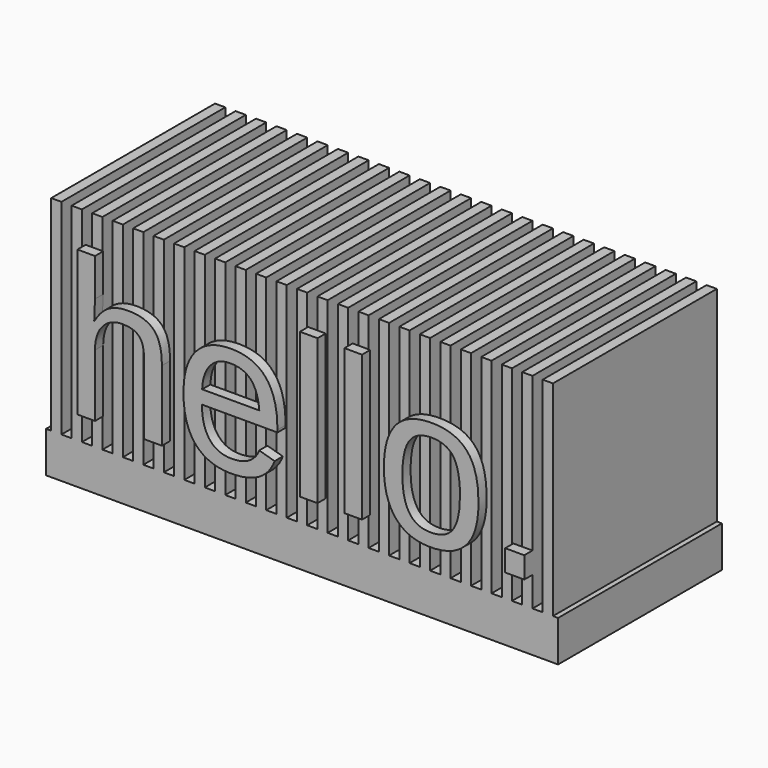
from build123d import *

# Parameters (mm, degrees)
F0_W         = 63.5
F0_H         = 25.4
F1_DEPTH     = 5.08
F2_W         = 1.27
F2_H         = 25.4
F3_DEPTH     = 25.4
F4_TEXT_SIZE = 24.8562691131
F5_DEPTH     = 1.27


# Not quite as in the source:
# - Text() gives the source's letters only with a copy of the font that has no kerning and outlines rounded to 1/6400 em; it was checked with that copy


with BuildPart() as f1:
    # F0 (on Top) → F1 (new body)
    with BuildSketch(Plane.XY):
        Rectangle(F0_W, F0_H)
    extrude(amount=F1_DEPTH)

    # F2 (on face) → F3 (join)
    with BuildSketch(Plane.XY.offset(5.08)):
        with Locations((-30.48, 0)):
            Rectangle(F2_W, F2_H)
        with Locations((-27.94, 0)):
            Rectangle(F2_W, F2_H)
        with Locations((-25.4, 0)):
            Rectangle(F2_W, F2_H)
        with Locations((-22.86, 0)):
            Rectangle(F2_W, F2_H)
        with Locations((-20.32, 0)):
            Rectangle(F2_W, F2_H)
        with Locations((-17.78, 0)):
            Rectangle(F2_W, F2_H)
        with Locations((-15.24, 0)):
            Rectangle(F2_W, F2_H)
        with Locations((-12.7, 0)):
            Rectangle(F2_W, F2_H)
        with Locations((-10.16, 0)):
            Rectangle(F2_W, F2_H)
        with Locations((-7.62, 0)):
            Rectangle(F2_W, F2_H)
        with Locations((-5.08, 0)):
            Rectangle(F2_W, F2_H)
        with Locations((-2.54, 0)):
            Rectangle(F2_W, F2_H)
        Rectangle(F2_W, F2_H)
        with Locations((2.54, 0)):
            Rectangle(F2_W, F2_H)
        with Locations((5.08, 0)):
            Rectangle(F2_W, F2_H)
        with Locations((7.62, 0)):
            Rectangle(F2_W, F2_H)
        with Locations((10.16, 0)):
            Rectangle(F2_W, F2_H)
        with Locations((12.7, 0)):
            Rectangle(F2_W, F2_H)
        with Locations((15.24, 0)):
            Rectangle(F2_W, F2_H)
        with Locations((17.78, 0)):
            Rectangle(F2_W, F2_H)
        with Locations((20.32, 0)):
            Rectangle(F2_W, F2_H)
        with Locations((22.86, 0)):
            Rectangle(F2_W, F2_H)
        with Locations((25.4, 0)):
            Rectangle(F2_W, F2_H)
        with Locations((27.94, 0)):
            Rectangle(F2_W, F2_H)
        with Locations((30.48, 0)):
            Rectangle(F2_W, F2_H)
    extrude(amount=F3_DEPTH)

    # F4 (on face) → F5 (join)
    with BuildSketch(Plane.XZ.offset(12.7)):
        with Locations((-28.575, 8.7549638843)):
            Text('hello.', F4_TEXT_SIZE, font='Arimo', text_align=(TextAlign.LEFT, TextAlign.BOTTOM))
    extrude(amount=F5_DEPTH)


solid = f1.part
